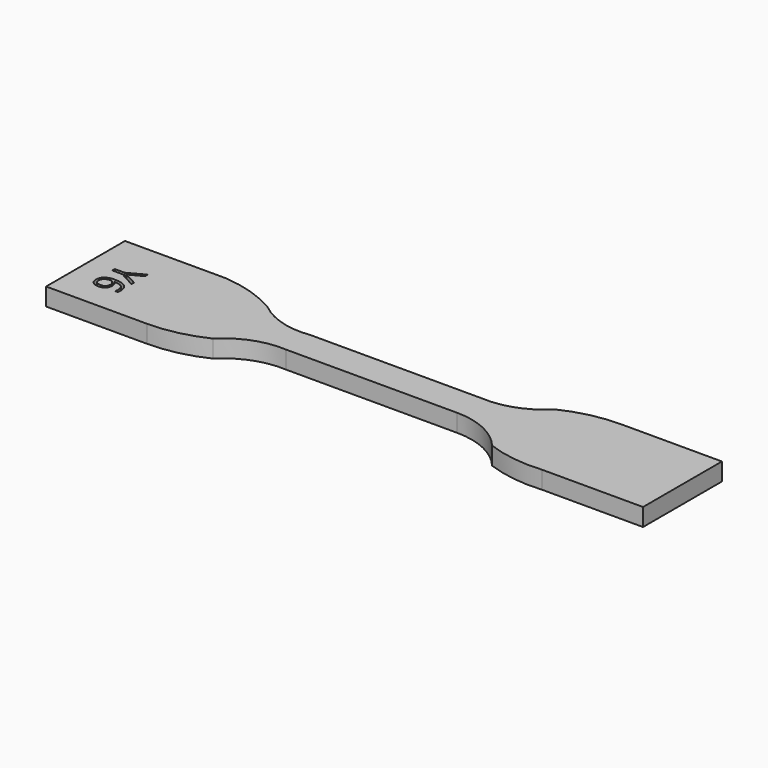
from build123d import *

# Parameters (mm, degrees)
F1_DEPTH     = 3.4
F2_TEXT_SIZE = 7.0564552314
F3_DEPTH     = 1


# Not quite as in the source:
# - Text() gives the source's letters only with a copy of the font that has no kerning and outlines rounded to 1/6400 em; it was checked with that copy


with BuildPart() as f1:
    # F0 (on Top) → F1 (new body)
    with BuildSketch(Plane.XY):
        with BuildLine():
            Line((-14.4320548165, 19.7811394548), (-33.8720548165, 19.7811394548))
            Line((-33.8720548165, 19.7811394548), (-33.8720548165, 0.7811394548))
            Line((-33.8720548165, 0.7811394548), (-14.4320548165, 0.7811394548))
            ThreePointArc((-14.4320548165, 0.7811394548), (-8.9053122052, 1.3996892086), (-3.6520548165, 3.2247301661))
            ThreePointArc((-3.6520548165, 3.2247301661), (1.3014698263, 6.4128780055), (7.1279451835, 7.2811394548))
            Line((7.1279451835, 7.2811394548), (40.1279451835, 7.2811394548))
            ThreePointArc((40.1279451835, 7.2811394548), (46.0837574042, 5.9511158081), (50.9079451835, 2.2137538538))
            ThreePointArc((50.9079451835, 2.2137538538), (56.2191047011, 0.9041953221), (61.6879451835, 0.7811394548))
            Line((61.6879451835, 0.7811394548), (81.1279451835, 0.7811394548))
            Line((81.1279451835, 0.7811394548), (81.1279451835, 19.7811394548))
            Line((81.1279451835, 19.7811394548), (61.6879451835, 19.7811394548))
            ThreePointArc((61.6879451835, 19.7811394548), (56.1612025723, 19.162589701), (50.9079451835, 17.3375487435))
            ThreePointArc((50.9079451835, 17.3375487435), (45.9544205407, 14.1494009041), (40.1279451835, 13.2811394548))
            Line((40.1279451835, 13.2811394548), (7.1279451835, 13.2811394548))
            ThreePointArc((7.1279451835, 13.2811394548), (1.4167452884, 13.6925537245), (-3.6520548165, 16.3560723447))
            ThreePointArc((-3.6520548165, 16.3560723447), (-8.8458057958, 18.686276846), (-14.4320548165, 19.7811394548))
        make_face()
    extrude(amount=F1_DEPTH)

    # F2 (on face) → F3 (cut)
    with BuildSketch(Plane.XY.offset(3.4)):
        with Locations(Location((-29.3720550835, 13.353464842), (0, 0, -90))):
            Text('Y6', F2_TEXT_SIZE, font='Open Sans', text_align=(TextAlign.LEFT, TextAlign.BOTTOM))
    extrude(amount=-F3_DEPTH, mode=Mode.SUBTRACT)


solid = f1.part
